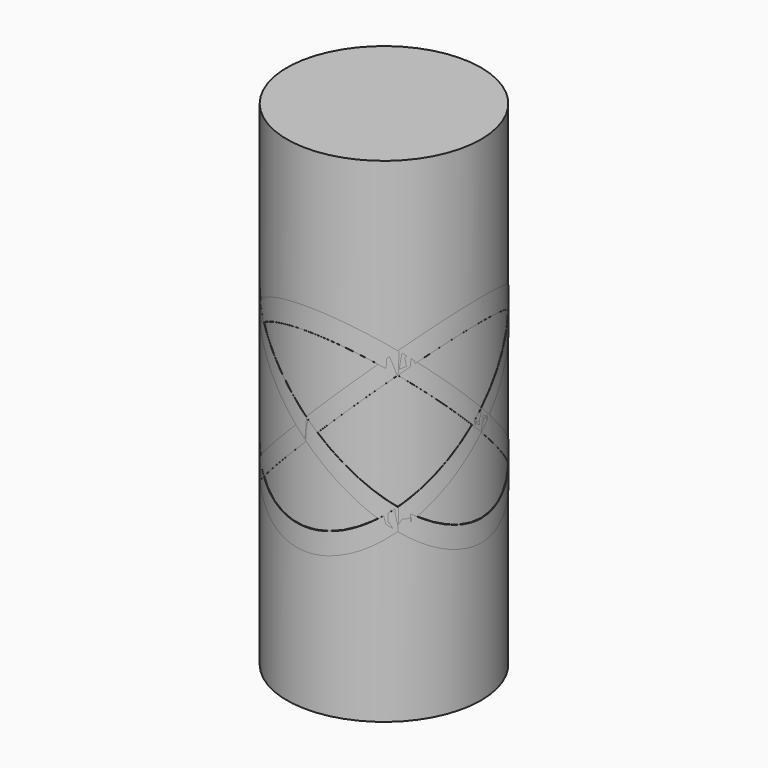
from build123d import *

# Parameters (mm, degrees)
F0_W          = 25.4
F0_H          = 25.4
F1_DEPTH      = 25.4
F3_DEPTH      = 12.7
F5_COUNT      = 4
F6_R          = 20.1833985855
F6_R_2        = 10.011648241
F7_DEPTH      = 25.401
F7_DEPTH_BACK = 25.401
F8_R          = 27.6664771381
F8_R_2        = 9.986248241
F9_DEPTH      = 50.801


with BuildPart() as f1:
    # F0 (on Top) → F1 (new body, symmetric)
    with BuildSketch(Plane.XY):
        Rectangle(F0_W, F0_H)
    extrude(amount=F1_DEPTH, both=True)


with BuildPart() as f3:
    # F2 (on Front) → F3 (new body, symmetric)
    with BuildSketch(Plane.XZ):
        Polygon((13.813551759, 12.7), (12.7, 13.813551759), (-11.1252, -10.011648241), (-10.011648241, -11.1252), align=None)
    extrude(amount=F3_DEPTH, both=True)


with BuildPart() as f5_1:
    # F5: instance of F3
    add(f3.part.rotate(Axis((0, 0, 26.6196299344), (0, 0, 1)), 1 * 360 / F5_COUNT))


with BuildPart() as f5_2:
    # F5: instance of F3
    add(f3.part.rotate(Axis((0, 0, 26.6196299344), (0, 0, 1)), 2 * 360 / F5_COUNT))


with BuildPart() as f5_3:
    # F5: instance of F3
    add(f3.part.rotate(Axis((0, 0, 26.6196299344), (0, 0, 1)), 3 * 360 / F5_COUNT))


with BuildPart() as f7_tool:
    # F6 (on Top) → F7 (new body, two sides)
    with BuildSketch(Plane.XY) as f7_sk:
        Circle(F6_R)
        Circle(F6_R_2, mode=Mode.SUBTRACT)
    extrude(amount=F7_DEPTH)
    extrude(f7_sk.sketch, amount=-F7_DEPTH_BACK)


with BuildPart() as f1_1:
    add(f1.part)

    # F7: cut by f7_tool
    add(f7_tool.part, mode=Mode.SUBTRACT)

    # F8 (on face) → F9 (cut, through all)
    with BuildSketch(Plane.XY.offset(25.4)):
        Circle(F8_R)
        Circle(F8_R_2, mode=Mode.SUBTRACT)
    extrude(amount=-F9_DEPTH, mode=Mode.SUBTRACT)


with BuildPart() as f3_1:
    add(f3.part)

    # F7: cut by f7_tool
    add(f7_tool.part, mode=Mode.SUBTRACT)


with BuildPart() as f5_1_1:
    add(f5_1.part)

    # F7: cut by f7_tool
    add(f7_tool.part, mode=Mode.SUBTRACT)


with BuildPart() as f5_2_1:
    add(f5_2.part)

    # F7: cut by f7_tool
    add(f7_tool.part, mode=Mode.SUBTRACT)


with BuildPart() as f5_3_1:
    add(f5_3.part)

    # F7: cut by f7_tool
    add(f7_tool.part, mode=Mode.SUBTRACT)


solid = Compound([f1_1.part, f3_1.part, f5_1_1.part, f5_2_1.part, f5_3_1.part])
